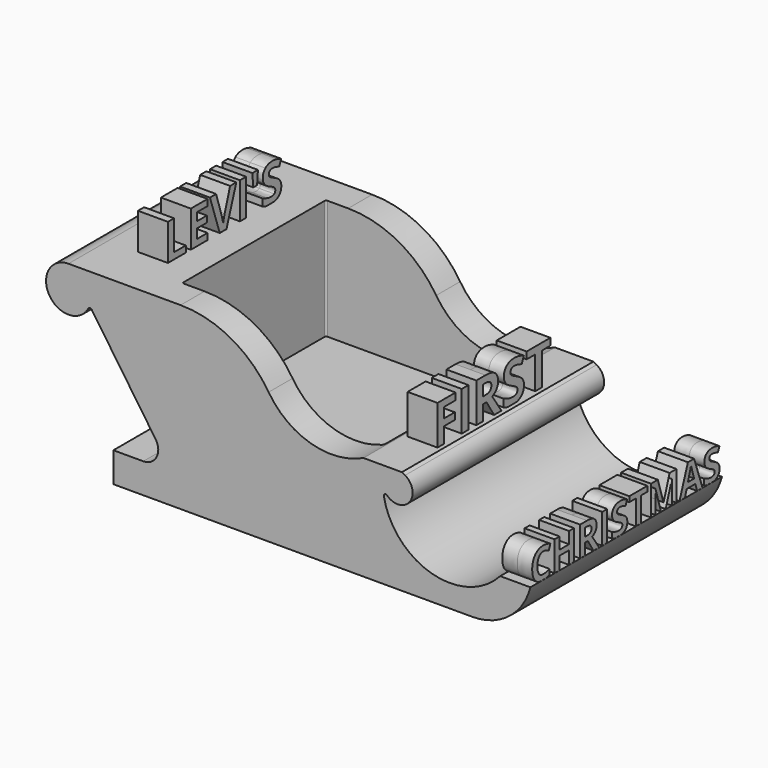
from build123d import *

# Parameters (mm, degrees)
F1_DEPTH      = 50.8
F3_DEPTH      = 50.8
F5_W          = 3.2611564554
F5_H          = 15.3769079924
F6_DEPTH      = 6.35
F9_TEXT_SIZE  = 23.3899280576
F10_DEPTH     = 6.35
F13_TEXT_SIZE = 17.723989424
F14_DEPTH     = 6.35


# Not quite as in the source:
# - Text() gives the source's letters only with a copy of the font that has no kerning and outlines rounded to 1/6400 em; it was checked with that copy


with BuildPart() as f1:
    # F0 (on Front) → F1 (new body, symmetric)
    with BuildSketch(Plane.XZ):
        with BuildLine():
            Line((-152.4, 12.7), (-152.4, 0))
            Line((-152.4, 0), (0, 0))
            ThreePointArc((0, 0), (15.5542598667, 5.3195368579), (24.5934442484, 19.05))
            Line((24.5934442484, 19.05), (11.7735474857, 19.05))
            ThreePointArc((11.7735474857, 19.05), (-17.2676670755, 10.5939691784), (-37.6334693878, 32.9575712278))
            ThreePointArc((-37.6334693878, 32.9575712278), (-37.2178568934, 33.8051744836), (-36.2857142857, 33.6559257524))
            ThreePointArc((-36.2857142857, 33.6559257524), (-26.7319957787, 34.2087105434), (-28.575, 43.599261314))
            ThreePointArc((-28.575, 43.599261314), (-29.2579773575, 43.9751591157), (-29.9557625579, 44.3227983575))
            Line((-29.9557625579, 44.3227983575), (-46.2442374421, 44.3227983575))
            ThreePointArc((-46.2442374421, 44.3227983575), (-68.5408487561, 42.4967536475), (-86.506806171, 55.8270833333))
            ThreePointArc((-86.506806171, 55.8270833333), (-102.5923642232, 70.7758174429), (-123.8711816931, 76.2))
            Line((-123.8711816931, 76.2), (-171.45, 76.2))
            ThreePointArc((-171.45, 76.2), (-179.603139061, 61.7503732678), (-163.0193088564, 62.2422726408))
            ThreePointArc((-163.0193088564, 62.2422726408), (-162.3630929223, 62.6652747523), (-161.6620423618, 62.321649593))
            Line((-161.6620423618, 62.321649593), (-134.4623288054, 22.6401671906))
            ThreePointArc((-134.4623288054, 22.6401671906), (-134.082168494, 16.0898531844), (-139.7, 12.7))
            Line((-139.7, 12.7), (-152.4, 12.7))
        make_face()
    extrude(amount=F1_DEPTH, both=True)

    # F2 (on face) → F3 (cut)
    with BuildSketch(Plane.XY.offset(76.2)):
        with BuildLine():
            Line((-123.8711816931, -38.1), (-123.8711816931, 38.1))
            Line((-123.8711816931, 38.1), (-132.55625, 38.1))
            ThreePointArc((-132.55625, 38.1), (-133.1175160076, 37.8675160076), (-133.35, 37.30625))
            Line((-133.35, 37.30625), (-133.35, -37.30625))
            ThreePointArc((-133.35, -37.30625), (-133.1175160076, -37.8675160076), (-132.55625, -38.1))
            Line((-132.55625, -38.1), (-123.8711816931, -38.1))
        make_face()
        with BuildLine():
            Line((-48.41875, 38.1), (-123.8711816931, 38.1))
            Line((-123.8711816931, 38.1), (-123.8711816931, -38.1))
            Line((-123.8711816931, -38.1), (-48.41875, -38.1))
            ThreePointArc((-48.41875, -38.1), (-47.8574839924, -37.8675160076), (-47.625, -37.30625))
            Line((-47.625, -37.30625), (-47.625, 37.30625))
            ThreePointArc((-47.625, 37.30625), (-47.8574839924, 37.8675160076), (-48.41875, 38.1))
        make_face()
    extrude(amount=-F3_DEPTH, mode=Mode.SUBTRACT)

    # F5 (on offset) → F6 (join, symmetric)
    with BuildSketch(Plane.YZ.offset(-152.4)):
        Polygon((-29.8148452406, 76.2), (-20.3174422302, 76.2), (-20.3174422302, 78.8923892304), (-26.5536887852, 78.8923892304), (-26.5536887852, 91.5769079924), (-29.8148452406, 91.5769079924), align=None)
        Polygon((-17.645245919, 76.2), (-8.7906508374, 76.2), (-8.7906508374, 78.8923892304), (-14.3840894636, 78.8923892304), (-14.3840894636, 82.8569323723), (-9.1776817893, 82.8569323723), (-9.1776817893, 85.5291286835), (-14.3840894636, 85.5291286835), (-14.3840894636, 88.9047116812), (-8.7906508374, 88.9047116812), (-8.7906508374, 91.5769079924), (-17.645245919, 91.5769079924), align=None)
        with BuildLine():
            Line((-2.301992792, 76.2), (1.2519609922, 76.2))
            Line((1.2519609922, 76.2), (6.4785615858, 91.5769079924))
            Line((6.4785615858, 91.5769079924), (3.1871157515, 91.5769079924))
            Line((3.1871157515, 91.5769079924), (0.2759698961, 82.4261500954))
            add(Edge.make_bspline(
                [(-0.5149194403, 79.0404706381), (-0.3971274115, 80.0063652745), (0.2759698961, 82.4261500954)],
                knots=[0, 0, 0, 1, 1, 1], degree=2))
            add(Edge.make_bspline(
                [(-0.8346406614, 80.5381121476), (-0.575498198, 79.4611564554), (-0.5149194403, 79.0404706381)],
                knots=[0, 0, 0, 1, 1, 1], degree=2))
            add(Edge.make_bspline(
                [(-1.3327326691, 82.4261500954), (-1.0937831249, 81.6150678397), (-0.8346406614, 80.5381121476)],
                knots=[0, 0, 0, 1, 1, 1], degree=2))
            Line((-1.3327326691, 82.4261500954), (-4.2270510918, 91.5769079924))
            Line((-4.2270510918, 91.5769079924), (-7.518496926, 91.5769079924))
            Line((-7.518496926, 91.5769079924), (-2.301992792, 76.2))
        make_face()
        with BuildLine():
            add(Edge.make_bspline(
                [(22.4624489712, 76.2), (21.3186583306, 76.4317594038), (20.3309041764, 76.9168486326)],
                knots=[0.477766543, 0.477766543, 0.477766543, 1, 1, 1], degree=2))
            Line((22.4624489712, 76.2), (26.7230090427, 76.2))
            add(Edge.make_bspline(
                [(28.853998834, 77.1877702989), (27.9849582783, 76.4923427835), (26.7230090427, 76.2)],
                knots=[0, 0, 0, 0.5796214889, 0.5796214889, 0.5796214889], degree=2))
            add(Edge.make_bspline(
                [(30.3533230867, 80.4708024168), (30.3533230867, 78.3875662497), (28.853998834, 77.1877702989)],
                knots=[0, 0, 0, 1, 1, 1], degree=2))
            add(Edge.make_bspline(
                [(29.5540200339, 83.0100620098), (30.3533230867, 81.9751748993), (30.3533230867, 80.4708024168)],
                knots=[0, 0, 0, 1, 1, 1], degree=2))
            add(Edge.make_bspline(
                [(26.5974401102, 85.0781534874), (28.7547169811, 84.0449491202), (29.5540200339, 83.0100620098)],
                knots=[0, 0, 0, 1, 1, 1], degree=2))
            add(Edge.make_bspline(
                [(24.5327141191, 86.1551091796), (24.9685446258, 85.8555808777), (26.5974401102, 85.0781534874)],
                knots=[0, 0, 0, 1, 1, 1], degree=2))
            add(Edge.make_bspline(
                [(23.8966371635, 86.7760414458), (24.0968836125, 86.4546374815), (24.5327141191, 86.1551091796)],
                knots=[0, 0, 0, 1, 1, 1], degree=2))
            add(Edge.make_bspline(
                [(23.6963907144, 87.5282276871), (23.6963907144, 87.0974454102), (23.8966371635, 86.7760414458)],
                knots=[0, 0, 0, 1, 1, 1], degree=2))
            add(Edge.make_bspline(
                [(24.1911172355, 88.6523001908), (23.6963907144, 88.2215179139), (23.6963907144, 87.5282276871)],
                knots=[0, 0, 0, 1, 1, 1], degree=2))
            add(Edge.make_bspline(
                [(25.6113525546, 89.0830824677), (24.6858437566, 89.0830824677), (24.1911172355, 88.6523001908)],
                knots=[0, 0, 0, 1, 1, 1], degree=2))
            add(Edge.make_bspline(
                [(27.1931312275, 88.8828360187), (26.3887799449, 89.0830824677), (25.6113525546, 89.0830824677)],
                knots=[0, 0, 0, 1, 1, 1], degree=2))
            add(Edge.make_bspline(
                [(29.229250583, 88.1777665889), (27.9974825101, 88.6825895696), (27.1931312275, 88.8828360187)],
                knots=[0, 0, 0, 1, 1, 1], degree=2))
            Line((29.229250583, 88.1777665889), (30.2792823829, 90.7153434386))
            add(Edge.make_bspline(
                [(28.0025307399, 91.5129637481), (29.0912656349, 91.2302628789), (30.2792823829, 90.7153434386)],
                knots=[0, 0, 0, 1, 1, 1], degree=2))
            add(Edge.make_bspline(
                [(25.7156826373, 91.7956646173), (26.9137958448, 91.7956646173), (28.0025307399, 91.5129637481)],
                knots=[0, 0, 0, 1, 1, 1], degree=2))
            add(Edge.make_bspline(
                [(21.89248993, 90.6295235319), (23.2757048972, 91.7956646173), (25.7156826373, 91.7956646173)],
                knots=[0, 0, 0, 1, 1, 1], degree=2))
            add(Edge.make_bspline(
                [(20.5092749629, 87.4205321179), (20.5092749629, 89.4633824465), (21.89248993, 90.6295235319)],
                knots=[0, 0, 0, 1, 1, 1], degree=2))
            add(Edge.make_bspline(
                [(20.9299607802, 85.5291286835), (20.5092749629, 86.3402109392), (20.5092749629, 87.4205321179)],
                knots=[0, 0, 0, 1, 1, 1], degree=2))
            add(Edge.make_bspline(
                [(22.0557160271, 84.1088933644), (21.3506465974, 84.7180464278), (20.9299607802, 85.5291286835)],
                knots=[0, 0, 0, 1, 1, 1], degree=2))
            add(Edge.make_bspline(
                [(24.1675588298, 82.836739453), (22.7607854569, 83.499740301), (22.0557160271, 84.1088933644)],
                knots=[0, 0, 0, 1, 1, 1], degree=2))
            add(Edge.make_bspline(
                [(26.1616096036, 81.7951213695), (25.6719313123, 82.1198908204), (24.1675588298, 82.836739453)],
                knots=[0, 0, 0, 1, 1, 1], degree=2))
            add(Edge.make_bspline(
                [(26.9036993852, 81.1169758321), (26.6512878948, 81.4703519186), (26.1616096036, 81.7951213695)],
                knots=[0, 0, 0, 1, 1, 1], degree=2))
            add(Edge.make_bspline(
                [(27.1561108756, 80.3126245495), (27.1561108756, 80.7635997456), (26.9036993852, 81.1169758321)],
                knots=[0, 0, 0, 1, 1, 1], degree=2))
            add(Edge.make_bspline(
                [(26.5822954208, 79.0926356795), (27.1561108756, 79.5015422938), (27.1561108756, 80.3126245495)],
                knots=[0, 0, 0, 1, 1, 1], degree=2))
            add(Edge.make_bspline(
                [(24.938255247, 78.6837290651), (26.0084799661, 78.6837290651), (26.5822954208, 79.0926356795)],
                knots=[0, 0, 0, 1, 1, 1], degree=2))
            add(Edge.make_bspline(
                [(22.9643973924, 78.9664299343), (24.0430358279, 78.6837290651), (24.938255247, 78.6837290651)],
                knots=[0, 0, 0, 1, 1, 1], degree=2))
            add(Edge.make_bspline(
                [(20.3309041764, 79.9457865169), (21.885758957, 79.2491308035), (22.9643973924, 78.9664299343)],
                knots=[0, 0, 0, 1, 1, 1], degree=2))
            Line((20.3309041764, 79.9457865169), (20.3309041764, 76.9168486326))
        make_face()
        with BuildLine():
            Line((26.7230090427, 76.2), (22.4624489712, 76.2))
            add(Edge.make_bspline(
                [(24.6858437566, 75.9879743481), (23.5088486088, 75.9879743481), (22.4624489712, 76.2)],
                knots=[0, 0, 0, 0.477766543, 0.477766543, 0.477766543], degree=2))
            add(Edge.make_bspline(
                [(26.7230090427, 76.2), (25.807762885, 75.9879743481), (24.6858437566, 75.9879743481)],
                knots=[0.5796214889, 0.5796214889, 0.5796214889, 1, 1, 1], degree=2))
        make_face()
        with Locations((10.0442945728, 83.8884539962)):
            Rectangle(F5_W, F5_H)
        Polygon((17.5106264575, 86.0238552046), (17.9447742209, 91.5769079924), (15.0100699597, 91.5769079924), (15.4408522366, 86.0238552046), align=None)
    extrude(amount=F6_DEPTH, both=True)

    # F9 (on face) → F10 (join, symmetric)
    with BuildSketch(Plane.YZ.offset(-38.1)):
        with Locations((-31.75, 44.3227983575)):
            Text('FIRST', F9_TEXT_SIZE, font='Open Sans', font_style=FontStyle.BOLD, text_align=(TextAlign.LEFT, TextAlign.BOTTOM))
    extrude(amount=F10_DEPTH, both=True)

    # F13 (on face) → F14 (join, symmetric)
    with BuildSketch(Plane.YZ.offset(18.1834958671)):
        with Locations((-50.8, 19.05)):
            Text('CHRISTMAS', F13_TEXT_SIZE, font='Open Sans', font_style=FontStyle.BOLD, text_align=(TextAlign.LEFT, TextAlign.BOTTOM))
    extrude(amount=F14_DEPTH, both=True)


solid = f1.part
